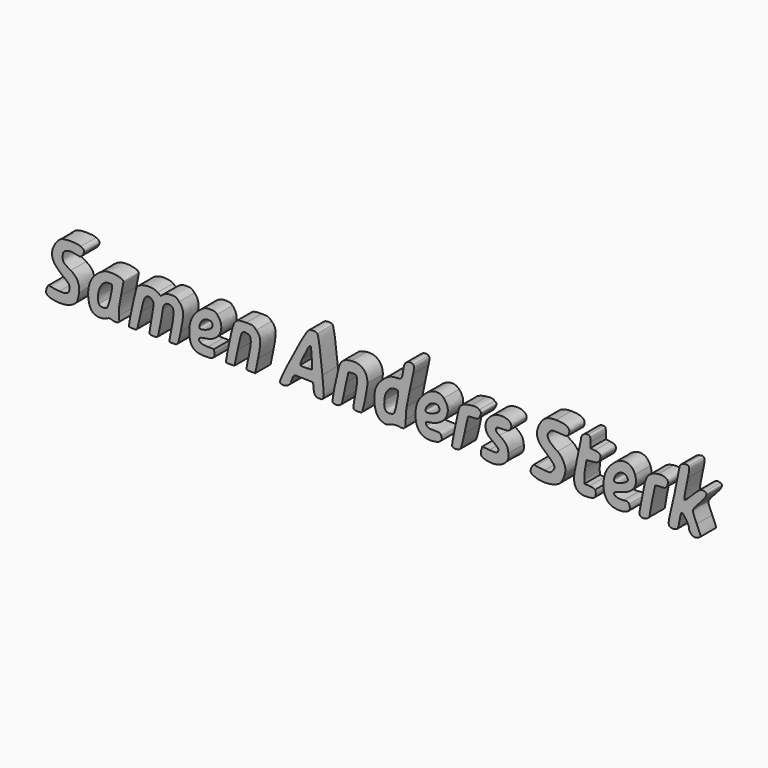
from build123d import *

# Parameters (mm, degrees)
F1_DEPTH = 50


# Not quite as in the source:
# - ends of sketch curves that miss each other by under 0.0002 mm in the source are joined


with BuildPart() as f1:
    # F0 (on Front) → F1 (new body)
    with BuildSketch(Plane.XZ):
        with BuildLine():
            add(Edge.make_bspline(
                [(-832.406244, -78.367915), (-856.572857, -74.842803), (-860.827692, -70.165915), (-854.65009, -53.917593)],
                knots=[0, 0, 0, 0, 1, 1, 1, 1], degree=3))
            add(Edge.make_bspline(
                [(-777.337056, -61.882833), (-786.075546, -75.21946), (-808.326543, -81.880345), (-832.406244, -78.367915)],
                knots=[0, 0, 0, 0, 1, 1, 1, 1], degree=3))
            add(Edge.make_bspline(
                [(-771.562903, -39.35764), (-772.263973, -48.091428), (-774.811041, -58.027653), (-777.337056, -61.882833)],
                knots=[0, 0, 0, 0, 1, 1, 1, 1], degree=3))
            add(Edge.make_bspline(
                [(-793.181698, 4.308785), (-776.337261, -5.306298), (-769.877008, -18.35494), (-771.562903, -39.35764)],
                knots=[0, 0, 0, 0, 1, 1, 1, 1], degree=3))
            add(Edge.make_bspline(
                [(-814.175385, 27.071832), (-814.175385, 17.848452), (-811.144725, 14.562372), (-793.181698, 4.308785)],
                knots=[0, 0, 0, 0, 1, 1, 1, 1], degree=3))
            add(Edge.make_bspline(
                [(-802.402596, 46.073807), (-812.066144, 42.884548), (-814.175385, 39.480108), (-814.175385, 27.071832)],
                knots=[0, 0, 0, 0, 1, 1, 1, 1], degree=3))
            add(Edge.make_bspline(
                [(-780.634888, 45.855009), (-790.500043, 48.22162), (-795.735208, 48.274242), (-802.402596, 46.073807)],
                knots=[0, 0, 0, 0, 1, 1, 1, 1], degree=3))
            add(Edge.make_bspline(
                [(-762.981328, 48.805224), (-767.454111, 42.988355), (-768.179811, 42.86708), (-780.634888, 45.855009)],
                knots=[0, 0, 0, 0, 1, 1, 1, 1], degree=3))
            add(Edge.make_bspline(
                [(-767.026528, 67.722129), (-757.027386, 63.544219), (-755.856898, 58.070571), (-762.981328, 48.805224)],
                knots=[0, 0, 0, 0, 1, 1, 1, 1], degree=3))
            add(Edge.make_bspline(
                [(-817.830584, 67.823566), (-806.684955, 72.480505), (-778.27919, 72.423791), (-767.026528, 67.722129)],
                knots=[0, 0, 0, 0, 1, 1, 1, 1], degree=3))
            add(Edge.make_bspline(
                [(-841.084753, 34.176215), (-838.413036, 47.534806), (-827.054827, 63.969432), (-817.830584, 67.823566)],
                knots=[0, 0, 0, 0, 1, 1, 1, 1], degree=3))
            add(Edge.make_bspline(
                [(-809.723088, -18.047695), (-836.259883, 2.215557), (-844.674467, 16.22765), (-841.084753, 34.176215)],
                knots=[0, 0, 0, 0, 1, 1, 1, 1], degree=3))
            add(Edge.make_bspline(
                [(-796.366198, -36.540753), (-796.366198, -29.526715), (-798.427288, -26.673063), (-809.723088, -18.047695)],
                knots=[0, 0, 0, 0, 1, 1, 1, 1], degree=3))
            add(Edge.make_bspline(
                [(-822.257235, -52.49464), (-803.083932, -53.938863), (-796.366198, -49.79944), (-796.366198, -36.540753)],
                knots=[0, 0, 0, 0, 1, 1, 1, 1], degree=3))
            add(Edge.make_bspline(
                [(-845.295043, -49.4374), (-841.472517, -50.452383), (-831.105504, -51.828145), (-822.257235, -52.49464)],
                knots=[0, 0, 0, 0, 1, 1, 1, 1], degree=3))
            add(Edge.make_bspline(
                [(-854.65009, -53.917593), (-852.609418, -48.550218), (-851.192246, -47.871528), (-845.295043, -49.4374)],
                knots=[0, 0, 0, 0, 1, 1, 1, 1], degree=3))
        make_face()
    extrude(amount=F1_DEPTH)


with BuildPart() as f1b:
    # F0 (on Front) → F1, piece 2 (new body)
    with BuildSketch(Plane.XZ):
        with BuildLine():
            add(Edge.make_bspline(
                [(13.269722, -77.429215), (1.650947, -72.380133), (-5.129428, -55.8634), (-5.129428, -32.609748)],
                knots=[0, 0, 0, 0, 1, 1, 1, 1], degree=3))
            add(Edge.make_bspline(
                [(38.223722, -77.389263), (25.075547, -82.028208), (23.857247, -82.030165), (13.269722, -77.429215)],
                knots=[0, 0, 0, 0, 1, 1, 1, 1], degree=3))
            add(Edge.make_bspline(
                [(57.403697, -75.086748), (52.563647, -74.178745), (44.620697, -75.132273), (38.223722, -77.389263)],
                knots=[0, 0, 0, 0, 1, 1, 1, 1], degree=3))
            add(Edge.make_bspline(
                [(76.394822, -53.720335), (76.270922, -75.590485), (73.958147, -78.192385), (57.403697, -75.086748)],
                knots=[0, 0, 0, 0, 1, 1, 1, 1], degree=3))
            add(Edge.make_bspline(
                [(78.673172, -23.99779), (77.481047, -29.594965), (76.455722, -42.970113), (76.394822, -53.720335)],
                knots=[0, 0, 0, 0, 1, 1, 1, 1], degree=3))
            add(Edge.make_bspline(
                [(86.162597, 12.892662), (83.235572, -1.799913), (79.865372, -18.400623), (78.673172, -23.99779)],
                knots=[0, 0, 0, 0, 1, 1, 1, 1], degree=3))
            add(Edge.make_bspline(
                [(95.491922, 57.165877), (93.287822, 47.508189), (89.089622, 27.585245), (86.162597, 12.892662)],
                knots=[0, 0, 0, 0, 1, 1, 1, 1], degree=3))
            add(Edge.make_bspline(
                [(95.739497, 78.485127), (99.056522, 75.168148), (99.027347, 72.657117), (95.491922, 57.165877)],
                knots=[0, 0, 0, 0, 1, 1, 1, 1], degree=3))
            add(Edge.make_bspline(
                [(75.373097, 75.222532), (81.326972, 81.17638), (91.429772, 82.79481), (95.739497, 78.485127)],
                knots=[0, 0, 0, 0, 1, 1, 1, 1], degree=3))
            add(Edge.make_bspline(
                [(69.787922, 56.781122), (70.763747, 64.827903), (73.277072, 73.126536), (75.373097, 75.222532)],
                knots=[0, 0, 0, 0, 1, 1, 1, 1], degree=3))
            add(Edge.make_bspline(
                [(50.880497, 33.825095), (65.975672, 34.168932), (67.230497, 35.6924), (69.787922, 56.781122)],
                knots=[0, 0, 0, 0, 1, 1, 1, 1], degree=3))
            add(Edge.make_bspline(
                [(12.167972, 13.688922), (26.489597, 28.443155), (36.193397, 33.490542), (50.880497, 33.825095)],
                knots=[0, 0, 0, 0, 1, 1, 1, 1], degree=3))
            add(Edge.make_bspline(
                [(-5.129428, -32.609748), (-5.129428, -11.483005), (-0.663928, 0.469422), (12.167972, 13.688922)],
                knots=[0, 0, 0, 0, 1, 1, 1, 1], degree=3))
        make_face()
        with BuildLine():
            add(Edge.make_bspline(
                [(45.610097, -49.612833), (50.044397, -44.269833), (59.227247, 2.981247), (56.383847, 5.824602)],
                knots=[0, 0, 0, 0, 1, 1, 1, 1], degree=3))
            add(Edge.make_bspline(
                [(34.083197, -53.25574), (38.760122, -53.25574), (43.947272, -51.616435), (45.610097, -49.612833)],
                knots=[0, 0, 0, 0, 1, 1, 1, 1], degree=3))
            add(Edge.make_bspline(
                [(20.827772, -27.497118), (19.439222, -46.694313), (22.815722, -53.25574), (34.083197, -53.25574)],
                knots=[0, 0, 0, 0, 1, 1, 1, 1], degree=3))
            add(Edge.make_bspline(
                [(45.697472, 7.353605), (32.665247, 6.069522), (22.194422, -8.60359), (20.827772, -27.497118)],
                knots=[0, 0, 0, 0, 1, 1, 1, 1], degree=3))
            add(Edge.make_bspline(
                [(56.383847, 5.824602), (55.091147, 7.117302), (50.282297, 7.80536), (45.697472, 7.353605)],
                knots=[0, 0, 0, 0, 1, 1, 1, 1], degree=3))
        make_face(mode=Mode.SUBTRACT)
    extrude(amount=F1_DEPTH)


with BuildPart() as f1c:
    # F0 (on Front) → F1, piece 3 (new body)
    with BuildSketch(Plane.XZ):
        with BuildLine():
            add(Edge.make_bspline(
                [(125.895347, -78.323658), (108.943247, -72.06469), (101.725697, -58.358275), (101.725697, -32.424385)],
                knots=[0, 0, 0, 0, 1, 1, 1, 1], degree=3))
            add(Edge.make_bspline(
                [(166.265822, -73.803933), (160.044572, -80.02525), (137.377322, -82.56298), (125.895347, -78.323658)],
                knots=[0, 0, 0, 0, 1, 1, 1, 1], degree=3))
            add(Edge.make_bspline(
                [(168.951797, -61.579218), (170.993522, -67.367268), (170.512322, -69.55747), (166.265822, -73.803933)],
                knots=[0, 0, 0, 0, 1, 1, 1, 1], degree=3))
            add(Edge.make_bspline(
                [(150.427247, -54.52783), (165.658247, -54.52783), (166.589447, -54.88231), (168.951797, -61.579218)],
                knots=[0, 0, 0, 0, 1, 1, 1, 1], degree=3))
            add(Edge.make_bspline(
                [(130.860272, -49.700718), (133.680122, -53.556903), (137.615822, -54.52783), (150.427247, -54.52783)],
                knots=[0, 0, 0, 0, 1, 1, 1, 1], degree=3))
            add(Edge.make_bspline(
                [(140.467922, -39.488283), (127.689497, -41.504523), (126.101222, -43.192735), (130.860272, -49.700718)],
                knots=[0, 0, 0, 0, 1, 1, 1, 1], degree=3))
            add(Edge.make_bspline(
                [(174.930272, 27.48269), (198.932372, 1.8596), (180.941522, -33.102183), (140.467922, -39.488283)],
                knots=[0, 0, 0, 0, 1, 1, 1, 1], degree=3))
            add(Edge.make_bspline(
                [(121.970972, 17.125737), (140.926172, 36.894009), (162.214472, 41.057239), (174.930272, 27.48269)],
                knots=[0, 0, 0, 0, 1, 1, 1, 1], degree=3))
            add(Edge.make_bspline(
                [(101.725697, -32.424385), (101.725697, -12.234858), (107.597147, 2.13539), (121.970972, 17.125737)],
                knots=[0, 0, 0, 0, 1, 1, 1, 1], degree=3))
        make_face()
        with BuildLine():
            add(Edge.make_bspline(
                [(148.386722, -16.110093), (162.021572, -11.464218), (166.936022, -5.038833), (162.785747, 2.715987)],
                knots=[0, 0, 0, 0, 1, 1, 1, 1], degree=3))
            add(Edge.make_bspline(
                [(129.503372, -9.280383), (125.084372, -20.903163), (129.564122, -22.523485), (148.386722, -16.110093)],
                knots=[0, 0, 0, 0, 1, 1, 1, 1], degree=3))
            add(Edge.make_bspline(
                [(162.785747, 2.715987), (157.070672, 13.39478), (135.115772, 5.48132), (129.503372, -9.280383)],
                knots=[0, 0, 0, 0, 1, 1, 1, 1], degree=3))
        make_face(mode=Mode.SUBTRACT)
    extrude(amount=F1_DEPTH)


with BuildPart() as f1d:
    # F0 (on Front) → F1, piece 4 (new body)
    with BuildSketch(Plane.XZ):
        with BuildLine():
            add(Edge.make_bspline(
                [(285.260522, -78.700788), (272.128547, -75.59827), (269.236922, -71.469363), (272.335922, -60.24568)],
                knots=[0, 0, 0, 0, 1, 1, 1, 1], degree=3))
            add(Edge.make_bspline(
                [(338.147522, -64.388087), (327.139247, -78.33514), (306.898547, -83.812863), (285.260522, -78.700788)],
                knots=[0, 0, 0, 0, 1, 1, 1, 1], degree=3))
            add(Edge.make_bspline(
                [(342.824897, -43.695542), (343.734047, -54.780438), (342.932822, -58.325335), (338.147522, -64.388087)],
                knots=[0, 0, 0, 0, 1, 1, 1, 1], degree=3))
            add(Edge.make_bspline(
                [(319.728722, -10.839895), (336.395897, -21.473448), (341.610872, -28.89199), (342.824897, -43.695542)],
                knots=[0, 0, 0, 0, 1, 1, 1, 1], degree=3))
            add(Edge.make_bspline(
                [(310.824122, 0.940505), (310.235072, -3.1993), (312.547247, -6.25816), (319.728722, -10.839895)],
                knots=[0, 0, 0, 0, 1, 1, 1, 1], degree=3))
            add(Edge.make_bspline(
                [(328.053722, 6.532242), (313.063997, 6.532242), (311.549822, 6.04082), (310.824122, 0.940505)],
                knots=[0, 0, 0, 0, 1, 1, 1, 1], degree=3))
            add(Edge.make_bspline(
                [(348.407072, 13.506755), (344.766197, 7.02785), (343.319897, 6.532242), (328.053722, 6.532242)],
                knots=[0, 0, 0, 0, 1, 1, 1, 1], degree=3))
            add(Edge.make_bspline(
                [(298.237772, 26.394162), (320.157197, 44.133939), (359.883497, 33.92909), (348.407072, 13.506755)],
                knots=[0, 0, 0, 0, 1, 1, 1, 1], degree=3))
            add(Edge.make_bspline(
                [(284.723372, -9.327078), (281.068847, 4.245012), (285.569672, 16.14161), (298.237772, 26.394162)],
                knots=[0, 0, 0, 0, 1, 1, 1, 1], degree=3))
            add(Edge.make_bspline(
                [(301.311572, -29.108665), (290.259122, -21.49654), (286.931897, -17.528808), (284.723372, -9.327078)],
                knots=[0, 0, 0, 0, 1, 1, 1, 1], degree=3))
            add(Edge.make_bspline(
                [(314.899247, -50.086195), (319.648847, -44.363268), (316.578872, -39.623673), (301.311572, -29.108665)],
                knots=[0, 0, 0, 0, 1, 1, 1, 1], degree=3))
            add(Edge.make_bspline(
                [(293.338022, -52.349485), (307.971497, -53.586468), (312.378197, -53.12389), (314.899247, -50.086195)],
                knots=[0, 0, 0, 0, 1, 1, 1, 1], degree=3))
            Line((293.338022, -52.349485), (274.945472, -50.794743))
            Line((274.945472, -50.794743), (272.335922, -60.24568))
        make_face()
    extrude(amount=F1_DEPTH)


with BuildPart() as f1e:
    # F0 (on Front) → F1, piece 5 (new body)
    with BuildSketch(Plane.XZ):
        with BuildLine():
            add(Edge.make_bspline(
                [(416.893397, -77.397992), (400.203422, -72.071747), (397.472222, -68.02945), (402.888797, -56.670768)],
                knots=[0, 0, 0, 0, 1, 1, 1, 1], degree=3))
            add(Edge.make_bspline(
                [(476.679722, -68.979723), (465.198122, -79.234525), (435.674597, -83.391618), (416.893397, -77.397992)],
                knots=[0, 0, 0, 0, 1, 1, 1, 1], degree=3))
            add(Edge.make_bspline(
                [(490.983647, -34.502628), (490.983647, -44.421902), (483.217772, -63.14026), (476.679722, -68.979723)],
                knots=[0, 0, 0, 0, 1, 1, 1, 1], degree=3))
            add(Edge.make_bspline(
                [(470.630297, 1.878897), (480.896522, -4.536385), (490.983647, -22.567068), (490.983647, -34.502628)],
                knots=[0, 0, 0, 0, 1, 1, 1, 1], degree=3))
            add(Edge.make_bspline(
                [(450.614597, 41.216163), (438.924872, 29.52641), (444.769997, 18.038788), (470.630297, 1.878897)],
                knots=[0, 0, 0, 0, 1, 1, 1, 1], degree=3))
            add(Edge.make_bspline(
                [(475.940072, 44.982577), (457.801247, 46.495297), (455.560472, 46.162049), (450.614597, 41.216163)],
                knots=[0, 0, 0, 0, 1, 1, 1, 1], degree=3))
            add(Edge.make_bspline(
                [(498.499997, 48.293941), (496.082597, 43.776936), (494.022497, 43.474559), (475.940072, 44.982577)],
                knots=[0, 0, 0, 0, 1, 1, 1, 1], degree=3))
            add(Edge.make_bspline(
                [(466.484072, 72.315294), (495.001172, 72.442325), (506.718722, 63.650719), (498.499997, 48.293941)],
                knots=[0, 0, 0, 0, 1, 1, 1, 1], degree=3))
            add(Edge.make_bspline(
                [(424.258622, 49.669334), (433.767422, 66.95015), (443.581022, 72.213274), (466.484072, 72.315294)],
                knots=[0, 0, 0, 0, 1, 1, 1, 1], degree=3))
            add(Edge.make_bspline(
                [(431.274347, -2.791757), (415.103597, 12.003688), (412.841297, 28.920005), (424.258622, 49.669334)],
                knots=[0, 0, 0, 0, 1, 1, 1, 1], degree=3))
            add(Edge.make_bspline(
                [(457.565972, -46.754095), (466.746647, -35.082843), (466.963547, -35.44558), (431.274347, -2.791757)],
                knots=[0, 0, 0, 0, 1, 1, 1, 1], degree=3))
            add(Edge.make_bspline(
                [(436.576622, -52.471165), (451.132172, -53.582965), (452.484047, -53.214752), (457.565972, -46.754095)],
                knots=[0, 0, 0, 0, 1, 1, 1, 1], degree=3))
            add(Edge.make_bspline(
                [(414.114422, -49.446093), (417.911972, -50.456297), (428.019947, -51.817585), (436.576622, -52.471165)],
                knots=[0, 0, 0, 0, 1, 1, 1, 1], degree=3))
            add(Edge.make_bspline(
                [(402.888797, -56.670768), (406.732247, -48.610998), (407.973122, -47.812382), (414.114422, -49.446093)],
                knots=[0, 0, 0, 0, 1, 1, 1, 1], degree=3))
        make_face()
    extrude(amount=F1_DEPTH)


with BuildPart() as f1f:
    # F0 (on Front) → F1, piece 6 (new body)
    with BuildSketch(Plane.XZ):
        with BuildLine():
            add(Edge.make_bspline(
                [(614.679422, -78.609858), (596.436647, -73.14775), (587.034272, -53.044368), (590.236847, -26.348883)],
                knots=[0, 0, 0, 0, 1, 1, 1, 1], degree=3))
            add(Edge.make_bspline(
                [(657.823322, -69.9157), (655.427372, -79.461768), (632.772347, -84.027108), (614.679422, -78.609858)],
                knots=[0, 0, 0, 0, 1, 1, 1, 1], degree=3))
            add(Edge.make_bspline(
                [(656.323697, -58.286095), (657.978047, -61.377235), (658.652822, -66.610555), (657.823322, -69.9157)],
                knots=[0, 0, 0, 0, 1, 1, 1, 1], degree=3))
            add(Edge.make_bspline(
                [(641.478347, -54.196795), (651.917372, -52.846705), (653.671172, -53.32981), (656.323697, -58.286095)],
                knots=[0, 0, 0, 0, 1, 1, 1, 1], degree=3))
            add(Edge.make_bspline(
                [(616.920047, -45.881523), (616.920047, -51.829593), (628.766822, -55.84081), (641.478347, -54.196795)],
                knots=[0, 0, 0, 0, 1, 1, 1, 1], degree=3))
            add(Edge.make_bspline(
                [(633.464372, -38.30914), (623.408897, -40.84039), (616.920047, -43.810368), (616.920047, -45.881523)],
                knots=[0, 0, 0, 0, 1, 1, 1, 1], degree=3))
            add(Edge.make_bspline(
                [(671.450222, 14.635167), (680.860547, -10.201315), (666.695972, -29.943745), (633.464372, -38.30914)],
                knots=[0, 0, 0, 0, 1, 1, 1, 1], degree=3))
            add(Edge.make_bspline(
                [(611.703047, 18.434667), (634.540847, 42.267994), (661.633247, 40.545108), (671.450222, 14.635167)],
                knots=[0, 0, 0, 0, 1, 1, 1, 1], degree=3))
            add(Edge.make_bspline(
                [(590.236847, -26.348883), (592.592897, -6.709833), (597.581522, 3.697565), (611.703047, 18.434667)],
                knots=[0, 0, 0, 0, 1, 1, 1, 1], degree=3))
        make_face()
        with BuildLine():
            add(Edge.make_bspline(
                [(639.660722, -15.16045), (653.289497, -9.318475), (656.225597, -4.169538), (649.908497, 2.810742)],
                knots=[0, 0, 0, 0, 1, 1, 1, 1], degree=3))
            add(Edge.make_bspline(
                [(619.775297, -6.61078), (612.793172, -21.252363), (619.111472, -23.968877), (639.660722, -15.16045)],
                knots=[0, 0, 0, 0, 1, 1, 1, 1], degree=3))
            add(Edge.make_bspline(
                [(649.908497, 2.810742), (641.526647, 12.07262), (626.434547, 7.353905), (619.775297, -6.61078)],
                knots=[0, 0, 0, 0, 1, 1, 1, 1], degree=3))
        make_face(mode=Mode.SUBTRACT)
    extrude(amount=F1_DEPTH)


with BuildPart() as f1g:
    # F0 (on Front) → F1, piece 7 (new body)
    with BuildSketch(Plane.XZ):
        with BuildLine():
            add(Edge.make_bspline(
                [(-735.872413, -72.960415), (-743.401618, -66.75187), (-747.859408, -52.093465), (-747.964775, -33.19756)],
                knots=[0, 0, 0, 0, 1, 1, 1, 1], degree=3))
            add(Edge.make_bspline(
                [(-699.684643, -74.879575), (-710.859936, -80.658543), (-727.614328, -79.770003), (-735.872413, -72.960415)],
                knots=[0, 0, 0, 0, 1, 1, 1, 1], degree=3))
            add(Edge.make_bspline(
                [(-686.005663, -73.93039), (-690.945665, -71.679573), (-693.891861, -71.884008), (-699.684643, -74.879575)],
                knots=[0, 0, 0, 0, 1, 1, 1, 1], degree=3))
            add(Edge.make_bspline(
                [(-673.044065, -75.126115), (-676.710118, -76.046238), (-682.542838, -75.508158), (-686.005663, -73.93039)],
                knots=[0, 0, 0, 0, 1, 1, 1, 1], degree=3))
            add(Edge.make_bspline(
                [(-667.993303, -58.90216), (-666.424738, -73.036645), (-666.569316, -73.501053), (-673.044065, -75.126115)],
                knots=[0, 0, 0, 0, 1, 1, 1, 1], degree=3))
            add(Edge.make_bspline(
                [(-663.022483, -11.985678), (-667.88963, -35.90563), (-669.186725, -48.14812), (-667.993303, -58.90216)],
                knots=[0, 0, 0, 0, 1, 1, 1, 1], degree=3))
            add(Edge.make_bspline(
                [(-656.43686, 22.931322), (-656.43686, 21.527982), (-659.400388, 5.815332), (-663.022483, -11.985678)],
                knots=[0, 0, 0, 0, 1, 1, 1, 1], degree=3))
            add(Edge.make_bspline(
                [(-687.614541, 33.24602), (-671.700403, 33.24602), (-656.43686, 28.196292), (-656.43686, 22.931322)],
                knots=[0, 0, 0, 0, 1, 1, 1, 1], degree=3))
            add(Edge.make_bspline(
                [(-715.20806, 25.998492), (-705.734811, 32.006247), (-701.014618, 33.24602), (-687.614541, 33.24602)],
                knots=[0, 0, 0, 0, 1, 1, 1, 1], degree=3))
            add(Edge.make_bspline(
                [(-747.964775, -33.19756), (-748.102146, -8.563173), (-736.42157, 12.545277), (-715.20806, 25.998492)],
                knots=[0, 0, 0, 0, 1, 1, 1, 1], degree=3))
        make_face()
        with BuildLine():
            add(Edge.make_bspline(
                [(-699.023173, -50.07553), (-694.75583, -46.829853), (-683.417135, 1.574795), (-685.960288, 5.689692)],
                knots=[0, 0, 0, 0, 1, 1, 1, 1], degree=3))
            add(Edge.make_bspline(
                [(-719.951593, -48.33466), (-716.91629, -54.006175), (-705.445611, -54.960333), (-699.023173, -50.07553)],
                knots=[0, 0, 0, 0, 1, 1, 1, 1], degree=3))
            add(Edge.make_bspline(
                [(-706.788223, 3.81995), (-719.650401, -5.189065), (-727.146748, -34.890385), (-719.951593, -48.33466)],
                knots=[0, 0, 0, 0, 1, 1, 1, 1], degree=3))
            add(Edge.make_bspline(
                [(-685.960288, 5.689692), (-688.129296, 9.199235), (-700.7222, 8.06876), (-706.788223, 3.81995)],
                knots=[0, 0, 0, 0, 1, 1, 1, 1], degree=3))
        make_face(mode=Mode.SUBTRACT)
    extrude(amount=F1_DEPTH)


with BuildPart() as f1h:
    # F0 (on Front) → F1, piece 8 (new body)
    with BuildSketch(Plane.XZ):
        with BuildLine():
            add(Edge.make_bspline(
                [(-467.340231, -74.98516), (-478.698065, -70.044753), (-483.32072, -61.60027), (-485.100441, -42.541465)],
                knots=[0, 0, 0, 0, 1, 1, 1, 1], degree=3))
            add(Edge.make_bspline(
                [(-423.931348, -75.404927), (-429.856191, -79.737265), (-457.019165, -79.4746), (-467.340231, -74.98516)],
                knots=[0, 0, 0, 0, 1, 1, 1, 1], degree=3))
            add(Edge.make_bspline(
                [(-420.264876, -63.320117), (-419.677445, -69.49579), (-420.76862, -73.09228), (-423.931348, -75.404927)],
                knots=[0, 0, 0, 0, 1, 1, 1, 1], degree=3))
            Line((-420.264876, -63.320117), (-421.101163, -54.52783))
            Line((-421.101163, -54.52783), (-437.01986, -54.419327))
            add(Edge.make_bspline(
                [(-457.08509, -50.164307), (-454.165453, -53.08393), (-448.228453, -54.342925), (-437.01986, -54.419327)],
                knots=[0, 0, 0, 0, 1, 1, 1, 1], degree=3))
            add(Edge.make_bspline(
                [(-443.949058, -37.253275), (-459.677473, -38.87659), (-464.062678, -43.186705), (-457.08509, -50.164307)],
                knots=[0, 0, 0, 0, 1, 1, 1, 1], degree=3))
            add(Edge.make_bspline(
                [(-413.125603, 27.521637), (-389.909848, 1.186272), (-406.355158, -33.373248), (-443.949058, -37.253275)],
                knots=[0, 0, 0, 0, 1, 1, 1, 1], degree=3))
            add(Edge.make_bspline(
                [(-431.355471, 33.24602), (-420.874911, 33.24602), (-417.137248, 32.072352), (-413.125603, 27.521637)],
                knots=[0, 0, 0, 0, 1, 1, 1, 1], degree=3))
            add(Edge.make_bspline(
                [(-456.155878, 24.37592), (-446.340021, 31.870895), (-442.495213, 33.24602), (-431.355471, 33.24602)],
                knots=[0, 0, 0, 0, 1, 1, 1, 1], degree=3))
            add(Edge.make_bspline(
                [(-485.100441, -42.541465), (-487.707021, -14.62837), (-478.075378, 7.639137), (-456.155878, 24.37592)],
                knots=[0, 0, 0, 0, 1, 1, 1, 1], degree=3))
        make_face()
        with BuildLine():
            add(Edge.make_bspline(
                [(-442.470208, -17.277108), (-430.028885, -13.098783), (-424.551088, -7.531263), (-425.43305, 0.039072)],
                knots=[0, 0, 0, 0, 1, 1, 1, 1], degree=3))
            add(Edge.make_bspline(
                [(-456.404293, -6.601968), (-462.817768, -20.05117), (-459.13388, -22.873473), (-442.470208, -17.277108)],
                knots=[0, 0, 0, 0, 1, 1, 1, 1], degree=3))
            add(Edge.make_bspline(
                [(-433.599043, 7.377132), (-443.791243, 8.539325), (-451.41131, 3.868392), (-456.404293, -6.601968)],
                knots=[0, 0, 0, 0, 1, 1, 1, 1], degree=3))
            add(Edge.make_bspline(
                [(-425.43305, 0.039072), (-426.022633, 5.099817), (-427.82408, 6.718625), (-433.599043, 7.377132)],
                knots=[0, 0, 0, 0, 1, 1, 1, 1], degree=3))
        make_face(mode=Mode.SUBTRACT)
    extrude(amount=F1_DEPTH)


with BuildPart() as f1i:
    # F0 (on Front) → F1, piece 9 (new body)
    with BuildSketch(Plane.XZ):
        with BuildLine():
            add(Edge.make_bspline(
                [(-249.222403, -76.298148), (-252.218721, -74.40235), (-248.616208, -65.431068), (-229.571443, -27.361848)],
                knots=[0, 0, 0, 0, 1, 1, 1, 1], degree=3))
            add(Edge.make_bspline(
                [(-221.323806, -65.01052), (-225.500106, -76.256207), (-240.010071, -82.126862), (-249.222403, -76.298148)],
                knots=[0, 0, 0, 0, 1, 1, 1, 1], degree=3))
            add(Edge.make_bspline(
                [(-188.958171, -46.166995), (-216.504583, -45.358607), (-213.341848, -43.51723), (-221.323806, -65.01052)],
                knots=[0, 0, 0, 0, 1, 1, 1, 1], degree=3))
            Line((-188.958171, -46.166995), (-164.140026, -46.89532))
            Line((-164.140026, -46.89532), (-162.783651, -60.397098))
            add(Edge.make_bspline(
                [(-147.278391, -78.65848), (-158.154613, -78.595105), (-161.331366, -74.853648), (-162.783651, -60.397098)],
                knots=[0, 0, 0, 0, 1, 1, 1, 1], degree=3))
            add(Edge.make_bspline(
                [(-139.840258, -22.267008), (-134.101933, -75.617028), (-134.512918, -78.732873), (-147.278391, -78.65848)],
                knots=[0, 0, 0, 0, 1, 1, 1, 1], degree=3))
            add(Edge.make_bspline(
                [(-153.365518, 68.228351), (-150.178746, 64.163058), (-146.461506, 39.291633), (-139.840258, -22.267008)],
                knots=[0, 0, 0, 0, 1, 1, 1, 1], degree=3))
            add(Edge.make_bspline(
                [(-177.114733, 66.956266), (-172.385323, 72.129756), (-157.067008, 72.950256), (-153.365518, 68.228351)],
                knots=[0, 0, 0, 0, 1, 1, 1, 1], degree=3))
            add(Edge.make_bspline(
                [(-229.571443, -27.361848), (-205.235698, 21.283685), (-184.058788, 59.360124), (-177.114733, 66.956266)],
                knots=[0, 0, 0, 0, 1, 1, 1, 1], degree=3))
        make_face()
        with BuildLine():
            add(Edge.make_bspline(
                [(-167.569385, 6.532242), (-168.05624, 20.525172), (-169.394728, 32.968962), (-170.543803, 34.185102)],
                knots=[0, 0, 0, 0, 1, 1, 1, 1], degree=3))
            Line((-167.569385, 6.532242), (-166.684198, -18.909453))
            Line((-166.684198, -18.909453), (-181.088698, -19.66576))
            add(Edge.make_bspline(
                [(-197.095881, -17.828853), (-196.214398, -19.25512), (-189.011166, -20.081733), (-181.088698, -19.66576)],
                knots=[0, 0, 0, 0, 1, 1, 1, 1], degree=3))
            add(Edge.make_bspline(
                [(-190.596921, 0.73664), (-195.052836, -8.04811), (-197.977378, -16.402585), (-197.095881, -17.828853)],
                knots=[0, 0, 0, 0, 1, 1, 1, 1], degree=3))
            add(Edge.make_bspline(
                [(-177.564163, 26.552592), (-180.276268, 21.138575), (-186.141013, 9.52139), (-190.596921, 0.73664)],
                knots=[0, 0, 0, 0, 1, 1, 1, 1], degree=3))
            add(Edge.make_bspline(
                [(-170.543803, 34.185102), (-171.692878, 35.401248), (-174.85205, 31.966617), (-177.564163, 26.552592)],
                knots=[0, 0, 0, 0, 1, 1, 1, 1], degree=3))
        make_face(mode=Mode.SUBTRACT)
    extrude(amount=F1_DEPTH)


with BuildPart() as f1j:
    # F0 (on Front) → F1, piece 10 (new body)
    with BuildSketch(Plane.XZ):
        with BuildLine():
            add(Edge.make_bspline(
                [(-113.552653, -75.027243), (-115.052728, -71.11798), (-104.465953, -16.19248), (-97.397653, 8.78645)],
                knots=[0, 0, 0, 0, 1, 1, 1, 1], degree=3))
            add(Edge.make_bspline(
                [(-93.355228, -75.517225), (-99.253828, -79.842708), (-111.821803, -79.53781), (-113.552653, -75.027243)],
                knots=[0, 0, 0, 0, 1, 1, 1, 1], degree=3))
            add(Edge.make_bspline(
                [(-86.504278, -58.344078), (-87.912178, -66.179778), (-90.926728, -73.736388), (-93.355228, -75.517225)],
                knots=[0, 0, 0, 0, 1, 1, 1, 1], degree=3))
            add(Edge.make_bspline(
                [(-78.086053, -18.909453), (-81.333253, -32.902383), (-85.121503, -50.647968), (-86.504278, -58.344078)],
                knots=[0, 0, 0, 0, 1, 1, 1, 1], degree=3))
            Line((-78.086053, -18.909453), (-72.181903, 6.532242))
            Line((-72.181903, 6.532242), (-62.991703, 7.311942))
            add(Edge.make_bspline(
                [(-53.594953, -33.7288), (-46.924678, 3.183995), (-48.157978, 8.570442), (-62.991703, 7.311942)],
                knots=[0, 0, 0, 0, 1, 1, 1, 1], degree=3))
            add(Edge.make_bspline(
                [(-49.953178, -75.69079), (-61.620178, -74.734345), (-61.420603, -77.034775), (-53.594953, -33.7288)],
                knots=[0, 0, 0, 0, 1, 1, 1, 1], degree=3))
            add(Edge.make_bspline(
                [(-37.660378, -74.083518), (-38.989678, -75.412803), (-44.521378, -76.13608), (-49.953178, -75.69079)],
                knots=[0, 0, 0, 0, 1, 1, 1, 1], degree=3))
            add(Edge.make_bspline(
                [(-22.951753, -2.90704), (-22.966753, -16.055508), (-34.255453, -70.6786), (-37.660378, -74.083518)],
                knots=[0, 0, 0, 0, 1, 1, 1, 1], degree=3))
            add(Edge.make_bspline(
                [(-64.926328, 34.627069), (-39.605503, 37.790698), (-22.920703, 22.870985), (-22.951753, -2.90704)],
                knots=[0, 0, 0, 0, 1, 1, 1, 1], degree=3))
            add(Edge.make_bspline(
                [(-97.397653, 8.78645), (-92.418028, 26.384172), (-85.251028, 32.087667), (-64.926328, 34.627069)],
                knots=[0, 0, 0, 0, 1, 1, 1, 1], degree=3))
        make_face()
    extrude(amount=F1_DEPTH)


with BuildPart() as f1k:
    # F0 (on Front) → F1, piece 11 (new body)
    with BuildSketch(Plane.XZ):
        with BuildLine():
            add(Edge.make_bspline(
                [(196.945622, -75.312738), (196.231247, -73.451148), (198.648947, -57.709105), (202.318322, -40.330405)],
                knots=[0, 0, 0, 0, 1, 1, 1, 1], degree=3))
            add(Edge.make_bspline(
                [(217.027247, -75.517225), (211.306697, -79.718155), (198.586472, -79.588623), (196.945622, -75.312738)],
                knots=[0, 0, 0, 0, 1, 1, 1, 1], degree=3))
            add(Edge.make_bspline(
                [(228.937697, -35.446555), (223.757672, -60.657265), (219.986747, -73.34389), (217.027247, -75.517225)],
                knots=[0, 0, 0, 0, 1, 1, 1, 1], degree=3))
            add(Edge.make_bspline(
                [(237.734372, 4.624115), (237.065147, 2.874995), (233.106647, -15.156805), (228.937697, -35.446555)],
                knots=[0, 0, 0, 0, 1, 1, 1, 1], degree=3))
            add(Edge.make_bspline(
                [(251.793047, 7.804325), (243.864647, 7.804325), (238.485647, 6.58754), (237.734372, 4.624115)],
                knots=[0, 0, 0, 0, 1, 1, 1, 1], degree=3))
            add(Edge.make_bspline(
                [(269.004422, 16.967375), (264.839522, 8.23343), (264.033497, 7.804325), (251.793047, 7.804325)],
                knots=[0, 0, 0, 0, 1, 1, 1, 1], degree=3))
            add(Edge.make_bspline(
                [(267.421097, 30.950787), (273.279497, 26.206917), (273.304697, 25.985022), (269.004422, 16.967375)],
                knots=[0, 0, 0, 0, 1, 1, 1, 1], degree=3))
            add(Edge.make_bspline(
                [(247.109297, 34.155305), (258.989597, 35.492224), (262.495772, 34.939061), (267.421097, 30.950787)],
                knots=[0, 0, 0, 0, 1, 1, 1, 1], degree=3))
            add(Edge.make_bspline(
                [(216.509297, 21.078162), (220.049222, 27.692615), (230.904647, 32.33174), (247.109297, 34.155305)],
                knots=[0, 0, 0, 0, 1, 1, 1, 1], degree=3))
            add(Edge.make_bspline(
                [(211.549997, 3.931355), (212.958122, 10.89662), (215.189822, 18.612687), (216.509297, 21.078162)],
                knots=[0, 0, 0, 0, 1, 1, 1, 1], degree=3))
            add(Edge.make_bspline(
                [(202.318322, -40.330405), (205.987697, -22.951713), (210.141947, -3.033918), (211.549997, 3.931355)],
                knots=[0, 0, 0, 0, 1, 1, 1, 1], degree=3))
        make_face()
    extrude(amount=F1_DEPTH)


with BuildPart() as f1l:
    # F0 (on Front) → F1, piece 12 (new body)
    with BuildSketch(Plane.XZ):
        with BuildLine():
            add(Edge.make_bspline(
                [(532.755572, -76.018083), (515.388047, -70.851588), (509.914697, -55.43566), (515.388647, -27.103533)],
                knots=[0, 0, 0, 0, 1, 1, 1, 1], degree=3))
            add(Edge.make_bspline(
                [(565.400672, -73.22413), (558.093797, -77.061475), (541.140497, -78.51244), (532.755572, -76.018083)],
                knots=[0, 0, 0, 0, 1, 1, 1, 1], degree=3))
            add(Edge.make_bspline(
                [(567.856697, -54.05515), (571.401347, -59.629623), (569.966822, -70.826095), (565.400672, -73.22413)],
                knots=[0, 0, 0, 0, 1, 1, 1, 1], degree=3))
            add(Edge.make_bspline(
                [(553.266647, -50.238895), (560.236097, -50.678568), (566.801522, -52.395888), (567.856697, -54.05515)],
                knots=[0, 0, 0, 0, 1, 1, 1, 1], degree=3))
            Line((553.266647, -50.238895), (540.594947, -49.439485))
            Line((540.594947, -49.439485), (539.921672, -39.26281))
            add(Edge.make_bspline(
                [(542.605097, -11.276943), (540.758822, -21.071995), (539.551322, -33.665635), (539.921672, -39.26281)],
                knots=[0, 0, 0, 0, 1, 1, 1, 1], degree=3))
            Line((542.605097, -11.276943), (545.961872, 6.532242))
            Line((545.961872, 6.532242), (560.569022, 7.84418))
            add(Edge.make_bspline(
                [(581.646722, 22.619577), (578.661047, 11.394485), (575.510747, 9.18617), (560.569022, 7.84418)],
                knots=[0, 0, 0, 0, 1, 1, 1, 1], degree=3))
            add(Edge.make_bspline(
                [(566.723297, 35.614797), (579.839447, 33.861417), (583.734722, 30.469467), (581.646722, 22.619577)],
                knots=[0, 0, 0, 0, 1, 1, 1, 1], degree=3))
            Line((566.723297, 35.614797), (555.859997, 37.067001))
            Line((555.859997, 37.067001), (555.859997, 51.05757))
            add(Edge.make_bspline(
                [(549.988547, 65.880405), (555.308297, 65.126337), (555.859997, 63.733625), (555.859997, 51.05757)],
                knots=[0, 0, 0, 0, 1, 1, 1, 1], degree=3))
            add(Edge.make_bspline(
                [(531.690422, 53.085314), (531.690422, 59.797441), (542.007422, 67.011706), (549.988547, 65.880405)],
                knots=[0, 0, 0, 0, 1, 1, 1, 1], degree=3))
            add(Edge.make_bspline(
                [(529.301597, 39.787075), (530.615447, 44.084302), (531.690422, 50.068509), (531.690422, 53.085314)],
                knots=[0, 0, 0, 0, 1, 1, 1, 1], degree=3))
            add(Edge.make_bspline(
                [(515.388647, -27.103533), (524.645672, 20.80907), (527.085497, 32.538897), (529.301597, 39.787075)],
                knots=[0, 0, 0, 0, 1, 1, 1, 1], degree=3))
        make_face()
    extrude(amount=F1_DEPTH)


with BuildPart() as f1m:
    # F0 (on Front) → F1, piece 13 (new body)
    with BuildSketch(Plane.XZ):
        with BuildLine():
            add(Edge.make_bspline(
                [(684.636347, -75.23761), (682.476197, -72.634765), (683.102372, -65.545248), (687.164297, -46.615698)],
                knots=[0, 0, 0, 0, 1, 1, 1, 1], degree=3))
            add(Edge.make_bspline(
                [(709.782272, -65.787775), (709.782272, -76.173123), (691.206347, -83.153958), (684.636347, -75.23761)],
                knots=[0, 0, 0, 0, 1, 1, 1, 1], degree=3))
            add(Edge.make_bspline(
                [(724.008872, 5.638287), (722.277272, 2.836415), (709.782272, -59.89573), (709.782272, -65.787775)],
                knots=[0, 0, 0, 0, 1, 1, 1, 1], degree=3))
            add(Edge.make_bspline(
                [(737.606747, 7.804325), (730.864247, 7.804325), (724.745147, 6.82961), (724.008872, 5.638287)],
                knots=[0, 0, 0, 0, 1, 1, 1, 1], degree=3))
            add(Edge.make_bspline(
                [(756.869072, 20.969885), (754.162997, 10.18796), (750.675572, 7.804325), (737.606747, 7.804325)],
                knots=[0, 0, 0, 0, 1, 1, 1, 1], degree=3))
            add(Edge.make_bspline(
                [(732.549197, 34.976885), (749.349272, 36.966603), (759.427172, 31.162227), (756.869072, 20.969885)],
                knots=[0, 0, 0, 0, 1, 1, 1, 1], degree=3))
            add(Edge.make_bspline(
                [(694.540322, -8.732778), (699.212447, 21.332967), (708.611522, 32.141825), (732.549197, 34.976885)],
                knots=[0, 0, 0, 0, 1, 1, 1, 1], degree=3))
            add(Edge.make_bspline(
                [(687.164297, -46.615698), (690.133922, -32.776563), (693.453122, -15.729243), (694.540322, -8.732778)],
                knots=[0, 0, 0, 0, 1, 1, 1, 1], degree=3))
        make_face()
    extrude(amount=F1_DEPTH)


with BuildPart() as f1n:
    # F0 (on Front) → F1, piece 14 (new body)
    with BuildSketch(Plane.XZ):
        with BuildLine():
            add(Edge.make_bspline(
                [(762.388997, -75.907578), (757.565672, -73.038648), (757.766972, -65.561568), (763.272947, -43.079065)],
                knots=[0, 0, 0, 0, 1, 1, 1, 1], degree=3))
            add(Edge.make_bspline(
                [(782.138747, -73.454223), (778.048772, -77.453853), (767.245022, -78.795925), (762.388997, -75.907578)],
                knots=[0, 0, 0, 0, 1, 1, 1, 1], degree=3))
            add(Edge.make_bspline(
                [(787.279472, -52.839408), (785.767547, -62.891118), (783.454247, -72.167778), (782.138747, -73.454223)],
                knots=[0, 0, 0, 0, 1, 1, 1, 1], degree=3))
            add(Edge.make_bspline(
                [(792.685397, -33.677913), (791.224022, -34.16503), (788.791322, -42.787698), (787.279472, -52.839408)],
                knots=[0, 0, 0, 0, 1, 1, 1, 1], degree=3))
            add(Edge.make_bspline(
                [(811.549022, -61.940208), (811.549022, -54.494013), (796.750847, -32.32276), (792.685397, -33.677913)],
                knots=[0, 0, 0, 0, 1, 1, 1, 1], degree=3))
            add(Edge.make_bspline(
                [(826.981322, -78.697435), (819.703397, -78.697435), (811.549022, -69.843003), (811.549022, -61.940208)],
                knots=[0, 0, 0, 0, 1, 1, 1, 1], degree=3))
            add(Edge.make_bspline(
                [(842.079122, -70.714263), (842.079122, -74.2501), (833.668322, -78.697435), (826.981322, -78.697435)],
                knots=[0, 0, 0, 0, 1, 1, 1, 1], degree=3))
            add(Edge.make_bspline(
                [(831.902447, -46.281985), (837.499622, -58.226043), (842.079122, -69.220563), (842.079122, -70.714263)],
                knots=[0, 0, 0, 0, 1, 1, 1, 1], degree=3))
            add(Edge.make_bspline(
                [(821.725697, -19.385935), (821.725697, -22.234713), (826.305272, -34.337935), (831.902447, -46.281985)],
                knots=[0, 0, 0, 0, 1, 1, 1, 1], degree=3))
            add(Edge.make_bspline(
                [(839.534897, 4.160337), (829.331672, -6.362343), (821.725697, -16.41844), (821.725697, -19.385935)],
                knots=[0, 0, 0, 0, 1, 1, 1, 1], degree=3))
            add(Edge.make_bspline(
                [(853.319747, 34.245905), (861.229697, 31.210587), (857.167547, 22.344935), (839.534897, 4.160337)],
                knots=[0, 0, 0, 0, 1, 1, 1, 1], degree=3))
            add(Edge.make_bspline(
                [(820.571147, 16.07525), (838.591022, 34.99273), (843.817097, 37.892424), (853.319747, 34.245905)],
                knots=[0, 0, 0, 0, 1, 1, 1, 1], degree=3))
            add(Edge.make_bspline(
                [(800.221922, -2.069973), (801.085322, -2.933313), (810.242447, 5.232035), (820.571147, 16.07525)],
                knots=[0, 0, 0, 0, 1, 1, 1, 1], degree=3))
            add(Edge.make_bspline(
                [(808.633547, 51.055207), (800.834897, 14.472807), (798.489797, -0.337848), (800.221922, -2.069973)],
                knots=[0, 0, 0, 0, 1, 1, 1, 1], degree=3))
            add(Edge.make_bspline(
                [(810.384872, 78.688656), (813.225422, 75.795716), (812.936747, 71.241258), (808.633547, 51.055207)],
                knots=[0, 0, 0, 0, 1, 1, 1, 1], degree=3))
            add(Edge.make_bspline(
                [(798.042647, 79.201641), (805.210022, 81.567098), (807.658547, 81.465334), (810.384872, 78.688656)],
                knots=[0, 0, 0, 0, 1, 1, 1, 1], degree=3))
            add(Edge.make_bspline(
                [(782.481722, 45.966868), (787.967222, 76.731499), (787.493672, 75.720174), (798.042647, 79.201641)],
                knots=[0, 0, 0, 0, 1, 1, 1, 1], degree=3))
            add(Edge.make_bspline(
                [(774.355397, 5.260152), (776.454572, 14.35556), (780.111422, 32.673582), (782.481722, 45.966868)],
                knots=[0, 0, 0, 0, 1, 1, 1, 1], degree=3))
            add(Edge.make_bspline(
                [(767.996222, -22.725708), (769.394597, -16.428888), (772.256297, -3.835248), (774.355397, 5.260152)],
                knots=[0, 0, 0, 0, 1, 1, 1, 1], degree=3))
            add(Edge.make_bspline(
                [(763.272947, -43.079065), (764.472347, -38.181535), (766.597772, -29.022528), (767.996222, -22.725708)],
                knots=[0, 0, 0, 0, 1, 1, 1, 1], degree=3))
        make_face()
    extrude(amount=F1_DEPTH)


with BuildPart() as f1o:
    # F0 (on Front) → F1, piece 15 (new body)
    with BuildSketch(Plane.XZ):
        with BuildLine():
            add(Edge.make_bspline(
                [(-641.695446, -74.78161), (-643.239605, -73.237458), (-639.15689, -51.199668), (-628.987948, -6.188605)],
                knots=[0, 0, 0, 0, 1, 1, 1, 1], degree=3))
            add(Edge.make_bspline(
                [(-630.742581, -76.15327), (-636.012246, -76.15327), (-640.941036, -75.53602), (-641.695446, -74.78161)],
                knots=[0, 0, 0, 0, 1, 1, 1, 1], degree=3))
            add(Edge.make_bspline(
                [(-610.925841, -31.69252), (-620.760861, -79.051825), (-619.468933, -76.15327), (-630.742581, -76.15327)],
                knots=[0, 0, 0, 0, 1, 1, 1, 1], degree=3))
            add(Edge.make_bspline(
                [(-590.196508, 10.348498), (-600.381711, 10.348498), (-603.514828, 3.99425), (-610.925841, -31.69252)],
                knots=[0, 0, 0, 0, 1, 1, 1, 1], degree=3))
            add(Edge.make_bspline(
                [(-581.287078, 5.153225), (-583.872995, 8.010628), (-587.882226, 10.348498), (-590.196508, 10.348498)],
                knots=[0, 0, 0, 0, 1, 1, 1, 1], degree=3))
            add(Edge.make_bspline(
                [(-583.185283, -36.189527), (-576.755451, -0.973202), (-576.706558, 0.09179), (-581.287078, 5.153225)],
                knots=[0, 0, 0, 0, 1, 1, 1, 1], degree=3))
            add(Edge.make_bspline(
                [(-588.614563, -74.245142), (-589.258371, -73.195667), (-586.815201, -56.070647), (-583.185283, -36.189527)],
                knots=[0, 0, 0, 0, 1, 1, 1, 1], degree=3))
            add(Edge.make_bspline(
                [(-577.465941, -76.15327), (-582.953863, -76.15327), (-587.970741, -75.29461), (-588.614563, -74.245142)],
                knots=[0, 0, 0, 0, 1, 1, 1, 1], degree=3))
            add(Edge.make_bspline(
                [(-566.183946, -70.428887), (-567.264021, -75.170582), (-569.200768, -76.15327), (-577.465941, -76.15327)],
                knots=[0, 0, 0, 0, 1, 1, 1, 1], degree=3))
            add(Edge.make_bspline(
                [(-554.131423, -6.26854), (-554.740806, -14.65762), (-560.671161, -46.227265), (-566.183946, -70.428887)],
                knots=[0, 0, 0, 0, 1, 1, 1, 1], degree=3))
            add(Edge.make_bspline(
                [(-533.281498, 8.375165), (-543.838783, 13.185395), (-553.195656, 6.613708), (-554.131423, -6.26854)],
                knots=[0, 0, 0, 0, 1, 1, 1, 1], degree=3))
            add(Edge.make_bspline(
                [(-526.728373, -8.042192), (-526.688923, 3.94304), (-527.385793, 5.688905), (-533.281498, 8.375165)],
                knots=[0, 0, 0, 0, 1, 1, 1, 1], degree=3))
            add(Edge.make_bspline(
                [(-530.710483, -39.26281), (-528.544633, -29.467757), (-526.752673, -15.41848), (-526.728373, -8.042192)],
                knots=[0, 0, 0, 0, 1, 1, 1, 1], degree=3))
            add(Edge.make_bspline(
                [(-536.089648, -66.612632), (-535.296958, -61.36528), (-532.876333, -49.057862), (-530.710483, -39.26281)],
                knots=[0, 0, 0, 0, 1, 1, 1, 1], degree=3))
            Line((-536.089648, -66.612632), (-537.530871, -76.15327))
            Line((-537.530871, -76.15327), (-526.964653, -76.15327))
            add(Edge.make_bspline(
                [(-507.460078, -41.806982), (-514.172361, -75.576287), (-514.500006, -76.15327), (-526.964653, -76.15327)],
                knots=[0, 0, 0, 0, 1, 1, 1, 1], degree=3))
            add(Edge.make_bspline(
                [(-511.808248, 24.395825), (-499.372723, 10.232578), (-498.812323, 1.699865), (-507.460078, -41.806982)],
                knots=[0, 0, 0, 0, 1, 1, 1, 1], degree=3))
            add(Edge.make_bspline(
                [(-532.139113, 33.24602), (-520.984506, 33.24602), (-518.709156, 32.255548), (-511.808248, 24.395825)],
                knots=[0, 0, 0, 0, 1, 1, 1, 1], degree=3))
            add(Edge.make_bspline(
                [(-552.228921, 27.679228), (-546.875736, 31.637015), (-541.069048, 33.24602), (-532.139113, 33.24602)],
                knots=[0, 0, 0, 0, 1, 1, 1, 1], degree=3))
            Line((-552.228921, 27.679228), (-559.758418, 22.112435))
            Line((-559.758418, 22.112435), (-567.287908, 27.679228))
            add(Edge.make_bspline(
                [(-613.18598, 28.789768), (-600.07142, 35.341231), (-576.892761, 34.780404), (-567.287908, 27.679228)],
                knots=[0, 0, 0, 0, 1, 1, 1, 1], degree=3))
            add(Edge.make_bspline(
                [(-628.987948, -6.188605), (-622.254643, 23.61515), (-621.878743, 24.447253), (-613.18598, 28.789768)],
                knots=[0, 0, 0, 0, 1, 1, 1, 1], degree=3))
        make_face()
    extrude(amount=F1_DEPTH)


with BuildPart() as f1p:
    # F0 (on Front) → F1, piece 16 (new body)
    with BuildSketch(Plane.XZ):
        with BuildLine():
            add(Edge.make_bspline(
                [(-389.961621, -74.380015), (-391.091923, -72.335733), (-387.293173, -52.19206), (-376.447963, -2.721145)],
                knots=[0, 0, 0, 0, 1, 1, 1, 1], degree=3))
            add(Edge.make_bspline(
                [(-378.353511, -75.652098), (-384.116691, -76.076102), (-389.340328, -75.503673), (-389.961621, -74.380015)],
                knots=[0, 0, 0, 0, 1, 1, 1, 1], degree=3))
            Line((-378.353511, -75.652098), (-367.875021, -74.88118))
            Line((-367.875021, -74.88118), (-359.949088, -36.241488))
            add(Edge.make_bspline(
                [(-348.724138, 6.373355), (-350.538636, 4.18703), (-355.589855, -14.989653), (-359.949088, -36.241488)],
                knots=[0, 0, 0, 0, 1, 1, 1, 1], degree=3))
            add(Edge.make_bspline(
                [(-330.615831, 7.714812), (-337.683891, 11.49752), (-344.916095, 10.961765), (-348.724138, 6.373355)],
                knots=[0, 0, 0, 0, 1, 1, 1, 1], degree=3))
            add(Edge.make_bspline(
                [(-330.572331, -39.26281), (-324.092661, -12.024782), (-324.107721, 4.231752), (-330.615831, 7.714812)],
                knots=[0, 0, 0, 0, 1, 1, 1, 1], degree=3))
            add(Edge.make_bspline(
                [(-336.278878, -67.248677), (-335.803326, -63.050793), (-333.235363, -50.457153), (-330.572331, -39.26281)],
                knots=[0, 0, 0, 0, 1, 1, 1, 1], degree=3))
            add(Edge.make_bspline(
                [(-325.704066, -74.88118), (-336.910648, -74.88118), (-337.125958, -74.725788), (-336.278878, -67.248677)],
                knots=[0, 0, 0, 0, 1, 1, 1, 1], degree=3))
            Line((-325.704066, -74.88118), (-314.264563, -74.88118))
            Line((-314.264563, -74.88118), (-306.928701, -38.877175))
            add(Edge.make_bspline(
                [(-311.648113, 24.796497), (-299.024473, 12.172865), (-298.358361, 3.185727), (-306.928701, -38.877175)],
                knots=[0, 0, 0, 0, 1, 1, 1, 1], degree=3))
            add(Edge.make_bspline(
                [(-337.525191, 33.23651), (-321.173331, 33.245435), (-319.576101, 32.724485), (-311.648113, 24.796497)],
                knots=[0, 0, 0, 0, 1, 1, 1, 1], degree=3))
            add(Edge.make_bspline(
                [(-376.447963, -2.721145), (-369.365526, 29.585787), (-365.430253, 33.221285), (-337.525191, 33.23651)],
                knots=[0, 0, 0, 0, 1, 1, 1, 1], degree=3))
        make_face()
    extrude(amount=F1_DEPTH)


solid = Compound([f1.part, f1b.part, f1c.part, f1d.part, f1e.part, f1f.part, f1g.part, f1h.part, f1i.part, f1j.part, f1k.part, f1l.part, f1m.part, f1n.part, f1o.part, f1p.part])
